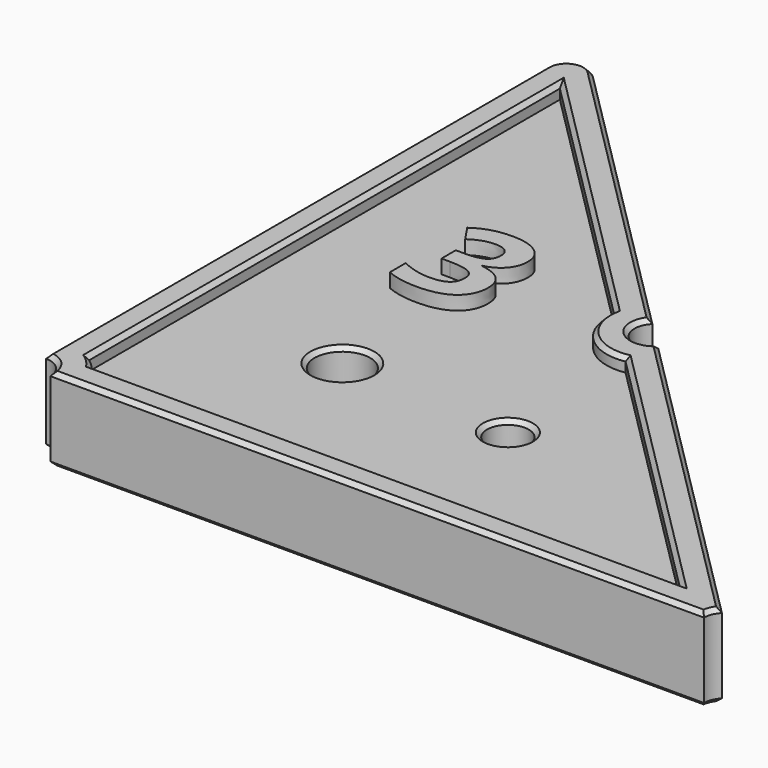
from build123d import *

# Parameters (mm, degrees)
F0_R         = 2
F0_R_2       = 1.5
F0_TEXT_SIZE = 11.1111111111
F1_DEPTH     = 5
F3_DEPTH     = 1
F4_SIZE      = 0.3


# Not quite as in the source:
# - Text() gives the source's letters only with a copy of the font that has no kerning and outlines rounded to 1/6400 em; it was checked with that copy


with BuildPart() as f1:
    # F0 (on Top) → F1 (new body)
    with BuildSketch(Plane.XY):
        with BuildLine():
            ThreePointArc((-22.4393398282, 22.4393398282), (-24.0740251485, 22.7644989552), (-25, 21.3786796564))
            Line((-25, 21.3786796564), (-25, -23.5))
            ThreePointArc((-25, -23.5), (-23.9393398282, -23.9393398282), (-23.5, -25))
            Line((-23.5, -25), (23.5, -25))
            ThreePointArc((23.5, -25), (23.6141807012, -24.4259748515), (23.9393398282, -23.9393398282))
            Line((23.9393398282, -23.9393398282), (1.0606601718, -1.0606601718))
            ThreePointArc((1.0606601718, -1.0606601718), (-1.0606601718, -1.0606601718), (-1.0606601718, 1.0606601718))
            Line((-1.0606601718, 1.0606601718), (-22.4393398282, 22.4393398282))
        make_face()
        with Locations((-12.5, -12.5)):
            Circle(F0_R, mode=Mode.SUBTRACT)
        with Locations((0, -13.25)):
            Circle(F0_R_2, mode=Mode.SUBTRACT)
        with BuildLine():
            add(Edge.make_bspline(
                [(-11.5998263889, 3.5460069444), (-10.8862847222, 3.046875), (-10.8862847222, 2.1579861111)],
                knots=[0, 0, 0, 1, 1, 1], degree=2))
            add(Edge.make_bspline(
                [(-10.8862847222, 2.1579861111), (-10.8862847222, 1.4149305556), (-11.3368055556, 0.8940972222)],
                knots=[0, 0, 0, 1, 1, 1], degree=2))
            add(Edge.make_bspline(
                [(-11.3368055556, 0.8940972222), (-11.7873263889, 0.3732638889), (-12.6015625, 0.1770833333)],
                knots=[0, 0, 0, 1, 1, 1], degree=2))
            Line((-12.6015625, 0.1770833333), (-12.6015625, 0.1458333333))
            add(Edge.make_bspline(
                [(-12.6015625, 0.1458333333), (-11.6397569444, 0.0260416667), (-11.1467013889, -0.4383680556)],
                knots=[0, 0, 0, 1, 1, 1], degree=2))
            add(Edge.make_bspline(
                [(-11.1467013889, -0.4383680556), (-10.6536458333, -0.9027777778), (-10.6536458333, -1.6892361111)],
                knots=[0, 0, 0, 1, 1, 1], degree=2))
            add(Edge.make_bspline(
                [(-10.6536458333, -1.6892361111), (-10.6536458333, -2.8333333333), (-11.4835069444, -3.4713541667)],
                knots=[0, 0, 0, 1, 1, 1], degree=2))
            add(Edge.make_bspline(
                [(-11.4835069444, -3.4713541667), (-12.3133680556, -4.109375), (-13.8532986111, -4.109375)],
                knots=[0, 0, 0, 1, 1, 1], degree=2))
            add(Edge.make_bspline(
                [(-13.8532986111, -4.109375), (-15.1449652778, -4.109375), (-16.1432291667, -3.6805555556)],
                knots=[0, 0, 0, 1, 1, 1], degree=2))
            Line((-16.1432291667, -3.6805555556), (-16.1432291667, -2.2534722222))
            add(Edge.make_bspline(
                [(-16.1432291667, -2.2534722222), (-15.6831597222, -2.4861111111), (-15.1293402778, -2.6328125)],
                knots=[0, 0, 0, 1, 1, 1], degree=2))
            add(Edge.make_bspline(
                [(-15.1293402778, -2.6328125), (-14.5755208333, -2.7795138889), (-14.0338541667, -2.7795138889)],
                knots=[0, 0, 0, 1, 1, 1], degree=2))
            add(Edge.make_bspline(
                [(-14.0338541667, -2.7795138889), (-13.2022569444, -2.7795138889), (-12.8064236111, -2.4973958333)],
                knots=[0, 0, 0, 1, 1, 1], degree=2))
            add(Edge.make_bspline(
                [(-12.8064236111, -2.4973958333), (-12.4105902778, -2.2152777778), (-12.4105902778, -1.5902777778)],
                knots=[0, 0, 0, 1, 1, 1], degree=2))
            add(Edge.make_bspline(
                [(-12.4105902778, -1.5902777778), (-12.4105902778, -1.0329861111), (-12.8663194444, -0.7994791667)],
                knots=[0, 0, 0, 1, 1, 1], degree=2))
            add(Edge.make_bspline(
                [(-12.8663194444, -0.7994791667), (-13.3220486111, -0.5659722222), (-14.3203125, -0.5659722222)],
                knots=[0, 0, 0, 1, 1, 1], degree=2))
            Line((-14.3203125, -0.5659722222), (-14.9227430556, -0.5659722222))
            Line((-14.9227430556, -0.5659722222), (-14.9227430556, 0.7204861111))
            Line((-14.9227430556, 0.7204861111), (-14.3098958333, 0.7204861111))
            add(Edge.make_bspline(
                [(-14.3098958333, 0.7204861111), (-13.3880208333, 0.7204861111), (-12.9618055556, 0.9618055556)],
                knots=[0, 0, 0, 1, 1, 1], degree=2))
            add(Edge.make_bspline(
                [(-12.9618055556, 0.9618055556), (-12.5355902778, 1.203125), (-12.5355902778, 1.7881944444)],
                knots=[0, 0, 0, 1, 1, 1], degree=2))
            add(Edge.make_bspline(
                [(-12.5355902778, 1.7881944444), (-12.5355902778, 2.6892361111), (-13.6640625, 2.6892361111)],
                knots=[0, 0, 0, 1, 1, 1], degree=2))
            add(Edge.make_bspline(
                [(-13.6640625, 2.6892361111), (-14.0546875, 2.6892361111), (-14.4592013889, 2.5590277778)],
                knots=[0, 0, 0, 1, 1, 1], degree=2))
            add(Edge.make_bspline(
                [(-14.4592013889, 2.5590277778), (-14.8637152778, 2.4288194444), (-15.3567708333, 2.109375)],
                knots=[0, 0, 0, 1, 1, 1], degree=2))
            Line((-15.3567708333, 2.109375), (-16.1328125, 3.2638888889))
            add(Edge.make_bspline(
                [(-16.1328125, 3.2638888889), (-15.0477430556, 4.0451388889), (-13.5442708333, 4.0451388889)],
                knots=[0, 0, 0, 1, 1, 1], degree=2))
            add(Edge.make_bspline(
                [(-13.5442708333, 4.0451388889), (-12.3133680556, 4.0451388889), (-11.5998263889, 3.5460069444)],
                knots=[0, 0, 0, 1, 1, 1], degree=2))
        make_face(mode=Mode.SUBTRACT)
        with Locations((-16.5668402778, -4)):
            Text('3', F0_TEXT_SIZE, font='Open Sans', font_style=FontStyle.BOLD, text_align=(TextAlign.LEFT, TextAlign.BOTTOM))
    extrude(amount=-F1_DEPTH)

    # F0 (on Top) + F2 (on face) → F3 (join)
    with BuildSketch(Plane.XY):
        with Locations((-16.5668402778, -4)):
            Text('3', F0_TEXT_SIZE, font='Open Sans', font_style=FontStyle.BOLD, text_align=(TextAlign.LEFT, TextAlign.BOTTOM))
    with BuildSketch(Plane.XY):
        with BuildLine():
            ThreePointArc((23.5, -25), (23.6141807012, -24.4259748515), (23.9393398282, -23.9393398282))
            Line((23.9393398282, -23.9393398282), (1.0606601718, -1.0606601718))
            ThreePointArc((1.0606601718, -1.0606601718), (-1.0606601718, -1.0606601718), (-1.0606601718, 1.0606601718))
            Line((-1.0606601718, 1.0606601718), (-22.4393398282, 22.4393398282))
            ThreePointArc((-22.4393398282, 22.4393398282), (-24.0740251485, 22.7644989552), (-25, 21.3786796564))
            Line((-25, 21.3786796564), (-25, -23.5))
            ThreePointArc((-25, -23.5), (-23.9393398282, -23.9393398282), (-23.5, -25))
            Line((-23.5, -25), (23.5, -25))
        make_face()
        with BuildLine():
            Line((0.616796011, -3.4452232522), (20.1715726765, -22.9999999177))
            Line((20.1715726765, -22.9999999177), (-22.1277186337, -22.9999999177))
            ThreePointArc((-22.1277186337, -22.9999999177), (-22.5251262076, -22.5251262076), (-22.9999999177, -22.1277186337))
            Line((-22.9999999177, -22.1277186337), (-22.9999999177, 20.1715726765))
            Line((-22.9999999177, 20.1715726765), (-3.4452232522, 0.616796011))
            ThreePointArc((-3.4452232522, 0.616796011), (-2.4748737924, -2.4748737924), (0.616796011, -3.4452232522))
        make_face(mode=Mode.SUBTRACT)
    extrude(amount=F3_DEPTH)

    # F4
    f4_edges = [f1.edges().sort_by_distance(p)[0] for p in [
        (-23.93934, -23.93934, 1),
        (0, -25, 1),
        (23.614181, -24.425975, 1),
        (12.5, -12.5, 1),
        (-1.06066, -1.06066, 1),
        (-11.75, 11.75, 1),
        (-24.074025, 22.764499, 1),
        (-25, -1.06066, 1),
        (10.394184, -13.222612, 1),
        (-0.978073, -23, 1),
        (-22.525126, -22.525126, 1),
        (-23, -0.978073, 1),
        (-13.222612, 10.394184, 1),
        (-2.474874, -2.474874, 1),
        (-14.5, -12.5, 0),
        (-1.5, -13.25, 0),
        (12.5, -12.5, -5),
        (-1.06066, -1.06066, -5),
        (-11.75, 11.75, -5),
        (-24.074025, 22.764499, -5),
        (-25, -1.06066, -5),
        (-23.93934, -23.93934, -5),
        (0, -25, -5),
        (23.614181, -24.425975, -5),
        (-14.5, -12.5, -5),
        (-1.5, -13.25, -5),
    ]]
    chamfer(f4_edges, length=F4_SIZE)


solid = f1.part
